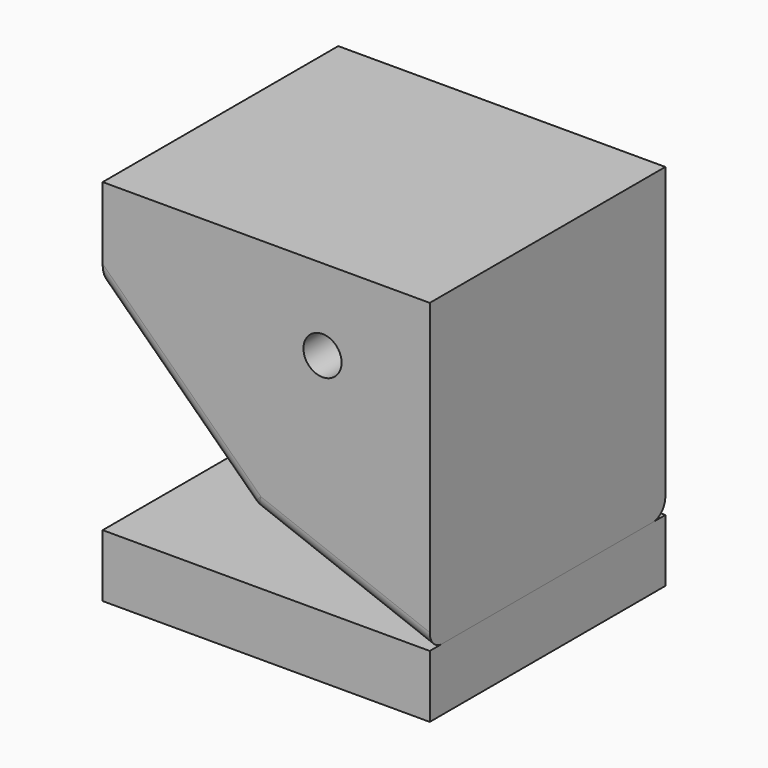
from build123d import *

# Parameters (mm, degrees)
F0_W         = 109.0031713247
F0_H         = 98.1307327747
F1_DEPTH     = 122.936
F3_DEPTH     = 228.6
F4_T1_DEPTH  = 81.2422372146
F4_T3_DEPTH  = 74.8836801522
F4_T5_DEPTH  = 87.9707327747
F4_T10_DEPTH = 5.08
F4_T16_DEPTH = 5.08
F6_D         = 12.7


# Not quite as in the source:
# - a fillet or chamfer that OpenCascade refuses, or shapes differently, is made with other operations: its cross-section is extruded or revolved along the edge and cut away or added


with BuildPart() as f1:
    # F0 (on Top) → F1 (new body)
    with BuildSketch(Plane.XY):
        Rectangle(F0_W, F0_H)
    extrude(amount=F1_DEPTH)

    # F2 (on face) → F3 (cut)
    with BuildSketch(Plane.XZ.offset(49.0653663874)):
        Polygon((-4.5534134842, 43.4030257165), (-54.5015856624, 91.8513536453), (-54.5015856624, 20.8180882037), (54.5015856624, 20.8180882037), align=None)
    extrude(amount=-F3_DEPTH, mode=Mode.SUBTRACT)

    # F4: fillet of radius 5.08 on 5 edges, made by hand

    # F4_s2 → F4_t1 (cut)
    with BuildSketch(Plane(origin=(-24.7859642555, 0, 24.0416910552), x_dir=(0, 1, 0), z_dir=(-0.7178017282, 0, 0.6962475702))):
        with BuildLine():
            ThreePointArc((49.0653663874, -33.0644637933), (47.5774688358, -29.4723613449), (43.9853663874, -27.9844637933))
            Line((43.9853663874, -27.9844637933), (49.0653663874, -27.9844637933))
            Line((49.0653663874, -27.9844637933), (49.0653663874, -33.0644637933))
        make_face()
        with BuildLine():
            ThreePointArc((-43.9853663874, -27.9844637933), (-47.5774688358, -29.4723613449), (-49.0653663874, -33.0644637933))
            Line((-49.0653663874, -33.0644637933), (-49.0653663874, -27.9844637933))
            Line((-49.0653663874, -27.9844637933), (-43.9853663874, -27.9844637933))
        make_face()
    extrude(amount=F4_T1_DEPTH, mode=Mode.SUBTRACT)

    # F4_s4 → F4_t3 (cut)
    with BuildSketch(Plane(origin=(52.4636836536, 0, -20.0641611063), x_dir=(0, 1, 0), z_dir=(-0.9340250041, 0, 0.3572076311))):
        with BuildLine():
            ThreePointArc((49.0653663874, -43.9929972277), (47.5774688358, -40.4008947793), (43.9853663874, -38.9129972277))
            Line((43.9853663874, -38.9129972277), (49.0653663874, -38.9129972277))
            Line((49.0653663874, -38.9129972277), (49.0653663874, -43.9929972277))
        make_face()
        with BuildLine():
            ThreePointArc((-43.9853663874, -38.9129972277), (-47.5774688358, -40.4008947793), (-49.0653663874, -43.9929972277))
            Line((-49.0653663874, -43.9929972277), (-49.0653663874, -38.9129972277))
            Line((-49.0653663874, -38.9129972277), (-43.9853663874, -38.9129972277))
        make_face()
    extrude(amount=F4_T3_DEPTH, mode=Mode.SUBTRACT)

    # F4_s6 → F4_t5 (cut)
    with BuildSketch(Plane.XZ.offset(-43.9853663874)):
        with BuildLine():
            ThreePointArc((-3.5795264455, 43.0305732869), (-4.4964692561, 43.4923147515), (-5.3018493359, 44.1289875285))
            Line((-5.3018493359, 44.1289875285), (-4.5534134842, 43.4030257165))
            Line((-4.5534134842, 43.4030257165), (-3.5795264455, 43.0305732869))
        make_face()
    extrude(amount=F4_T5_DEPTH, mode=Mode.SUBTRACT)


with BuildPart() as f4_tool8:
    # F4_s9 → F4_t10 (new body)
    with BuildSketch(Plane.XZ.offset(-43.9853663874)):
        Polygon((-1.7649116793, 47.7754203077), (-3.5795264455, 43.0305732869), (-4.5534134842, 43.4030257165), (-5.3018493359, 44.1289875285), align=None)
    extrude(amount=-F4_T10_DEPTH)

    # F4_s11 → F4_t12 (revolve, cut)
    with BuildSketch(Plane(origin=(-1.7649116793, 43.9853663874, 47.7754203077), x_dir=(0.5377081844, 0, 0.843131015), z_dir=(-0.843131015, 0, 0.5377081844))):
        with BuildLine():
            ThreePointArc((0, -5.08), (5.08, 0), (0, 5.08))
            Line((0, 5.08), (0, -5.08))
        make_face()
    revolve(axis=Axis((-1.7649116793, 43.9853663874, 47.7754203077), (0, 1, 0)), mode=Mode.SUBTRACT)


with BuildPart() as f1_1:
    add(f1.part)

    # F4_t7: cut F4_tool8
    add(f4_tool8.part, mode=Mode.SUBTRACT)


with BuildPart() as f4_tool14:
    # F4_s15 → F4_t16 (new body)
    with BuildSketch(Plane.XZ.offset(43.9853663874)):
        Polygon((-1.7649116793, 47.7754203077), (-3.5795264455, 43.0305732869), (-4.5534134842, 43.4030257165), (-5.3018493359, 44.1289875285), align=None)
    extrude(amount=F4_T16_DEPTH)

    # F4_s17 → F4_t18 (revolve, cut)
    with BuildSketch(Plane(origin=(-1.7649116793, -43.9853663874, 47.7754203077), x_dir=(0.5377081844, 0, 0.843131015), z_dir=(0.843131015, 0, -0.5377081844))):
        with BuildLine():
            ThreePointArc((0, -5.08), (5.08, 0), (0, 5.08))
            Line((0, 5.08), (0, -5.08))
        make_face()
    revolve(axis=Axis((-1.7649116793, -43.9853663874, 47.7754203077), (0, -1, 0)), mode=Mode.SUBTRACT)


with BuildPart() as f1_2:
    add(f1_1.part)

    # F4_t13: cut F4_tool14
    add(f4_tool14.part, mode=Mode.SUBTRACT)

    # F6 (through all)
    with Locations(Plane.XZ.offset(49.0653663874)):
        with Locations((18.7600683421, 95.8583652973)):
            Hole(F6_D / 2)


solid = f1_2.part
